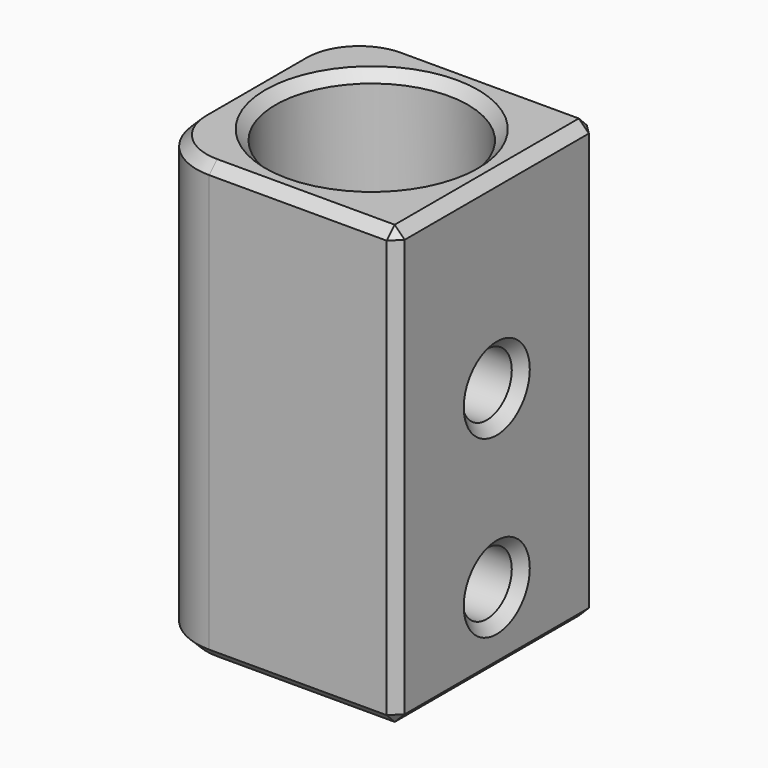
from build123d import *

# Parameters (mm, degrees)
F0_W           = 20
F0_H           = 20
F1_DEPTH       = 35
F2_R           = 7.7
F3_DEPTH       = 8.5
F5_D           = 5
F5_CSINK_D     = 9.8
F5_CSINK_ANGLE = 90
F6_R           = 5
F7_SIZE        = 0.8


with BuildPart() as f1:
    # F0 (on Top) → F1 (new body)
    with BuildSketch(Plane.XY):
        Rectangle(F0_W, F0_H)
    extrude(amount=F1_DEPTH)

    # F2 (on face) → F3 (cut)
    with BuildSketch(Plane.XY.offset(35)):
        Circle(F2_R)
    extrude(amount=-F3_DEPTH, mode=Mode.SUBTRACT)

    # F5 (through all)
    with Locations(Plane(origin=(-10, 0, 0), x_dir=(0, -1, 0), z_dir=(-1, 0, 0))):
        with Locations((0, 6), (0, 20)):
            CounterSinkHole(F5_D / 2, F5_CSINK_D / 2, counter_sink_angle=F5_CSINK_ANGLE)

    # F6
    f6_edges = [f1.edges().sort_by_distance(p)[0] for p in [
        (-10, -10, 17.5),
        (-10, 10, 17.5),
    ]]
    fillet(f6_edges, radius=F6_R)

    # F7
    f7_edges = [f1.edges().sort_by_distance(p)[0] for p in [
        (-7.7, 0, 35),
        (10, -10, 17.5),
        (10, 10, 17.5),
        (2.5, 10, 35),
        (-10, 0, 35),
        (10, 0, 35),
        (-10, 0, 0),
        (2.5, 10, 0),
        (10, 0, 0),
        (2.5, -10, 0),
        (2.5, -10, 35),
        (-8.535534, -8.535534, 0),
        (-8.535534, 8.535534, 0),
        (-8.535534, -8.535534, 35),
        (10, 2.5, 20),
        (10, 2.5, 6),
        (-8.535534, 8.535534, 35),
    ]]
    chamfer(f7_edges, length=F7_SIZE)


solid = f1.part
